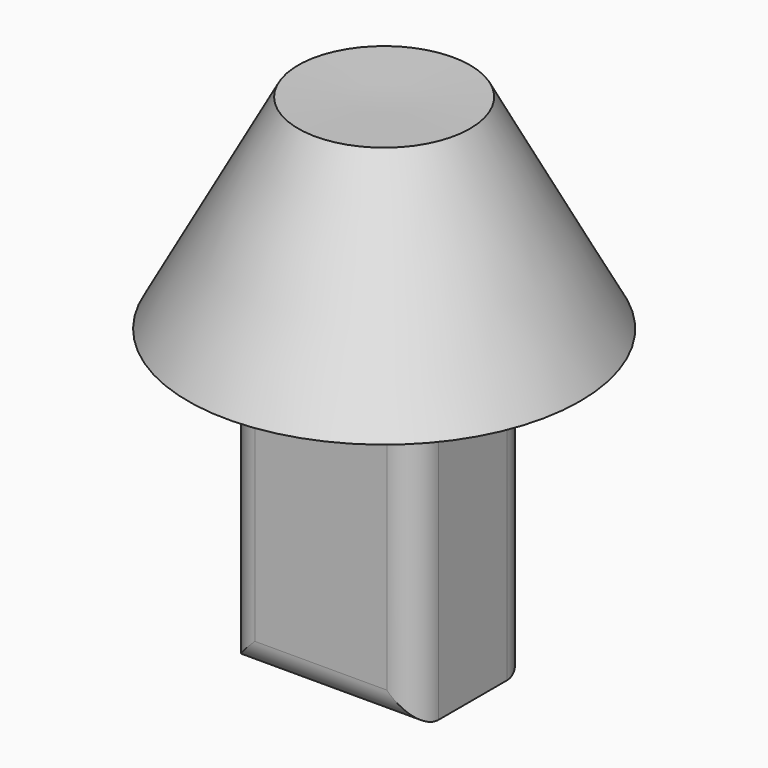
from build123d import *

# Parameters (mm, degrees)
F2_W         = 33.0171785317
F2_H         = 49.6530286036
F3_DEPTH     = 12.5
F4_R         = 5
F5_R         = 5
F6_T1_DEPTH  = 57.1530286036
F6_T3_DEPTH  = 58.0171785317
F6_T5_DEPTH  = 15
F6_S9_W      = 5
F6_S9_H      = 5
F6_T10_DEPTH = 5
F6_S15_W     = 5
F6_S15_H     = 5
F6_T16_DEPTH = 5
F6_T20_ANGLE = 90
F6_T22_ANGLE = 90


# Not quite as in the source:
# - a fillet or chamfer that OpenCascade refuses, or shapes differently, is made with other operations: its cross-section is extruded or revolved along the edge and cut away or added


with BuildPart() as f1:
    # F0 (on Front) → F1 (revolve)
    with BuildSketch(Plane.XZ):
        Polygon((10.2449354299, 42.7789126646), (10.2449354299, 7.6398269811), (44.4469846271, 7.6398269811), (25.2376164656, 43.2474373302), align=None)
    revolve(axis=Axis((10.2449354299, 0, 25.2093698228), (0, 0, 1)))


with BuildPart() as f3:
    # F2 (on Front) → F3 (new body, symmetric)
    with BuildSketch(Plane.XZ):
        with Locations((9.1960497666, -19.5281591732)):
            Rectangle(F2_W, F2_H)
    extrude(amount=F3_DEPTH, both=True)

    # F4
    f4_edges = [f3.edges().sort_by_distance(p)[0] for p in [
        (9.19605, 12.5, 5.298355),
    ]]
    fillet(f4_edges, radius=F4_R)

    # F5
    f5_edges = [f3.edges().sort_by_distance(p)[0] for p in [
        (9.19605, -12.5, 5.298355),
        (-7.312539, -12.5, -19.528159),
        (9.19605, -12.5, -44.354673),
        (25.704639, -12.5, -19.528159),
    ]]
    fillet(f5_edges, radius=F5_R)

    # F6: fillet of radius 5 on 4 edges, made by hand

    # F6_s2 → F6_t1 (cut)
    with BuildSketch(Plane.XY.offset(-56.854673475)):
        with BuildLine():
            ThreePointArc((-7.3125394993, 7.5), (-5.8480734052, 11.0355339059), (-2.3125394993, 12.5))
            Line((-2.3125394993, 12.5), (-7.3125394993, 12.5))
            Line((-7.3125394993, 12.5), (-7.3125394993, 7.5))
        make_face()
        with BuildLine():
            ThreePointArc((25.7046390325, 7.5), (24.2401729384, 11.0355339059), (20.7046390325, 12.5))
            Line((20.7046390325, 12.5), (25.7046390325, 12.5))
            Line((25.7046390325, 12.5), (25.7046390325, 7.5))
        make_face()
    extrude(amount=F6_T1_DEPTH, mode=Mode.SUBTRACT)

    # F6_s4 → F6_t3 (cut)
    with BuildSketch(Plane.YZ.offset(-19.8125394993)):
        with BuildLine():
            ThreePointArc((7.5, -44.354673475), (11.0355339059, -42.890207381), (12.5, -39.354673475))
            Line((12.5, -39.354673475), (12.5, -44.354673475))
            Line((12.5, -44.354673475), (7.5, -44.354673475))
        make_face()
    extrude(amount=F6_T3_DEPTH, mode=Mode.SUBTRACT)

    # F6_s6 → F6_t5 (cut)
    with BuildSketch(Plane.XZ.offset(-7.5)):
        with BuildLine():
            ThreePointArc((20.7046390325, 5.2983551286), (24.2401729384, 3.8338890345), (25.7046390325, 0.2983551286))
            Line((25.7046390325, 0.2983551286), (25.7046390325, 5.2983551286))
            Line((25.7046390325, 5.2983551286), (20.7046390325, 5.2983551286))
        make_face()
        with BuildLine():
            ThreePointArc((-2.3125394993, 5.2983551286), (-5.8480734052, 3.8338890345), (-7.3125394993, 0.2983551286))
            Line((-7.3125394993, 0.2983551286), (-7.3125394993, 5.2983551286))
            Line((-7.3125394993, 5.2983551286), (-2.3125394993, 5.2983551286))
        make_face()
    extrude(amount=F6_T5_DEPTH, mode=Mode.SUBTRACT)


with BuildPart() as f6_tool8:
    # F6_s9 → F6_t10 (new body)
    with BuildSketch(Plane.XY.offset(0.2983551286)):
        with Locations((23.2046390325, -10)):
            Rectangle(F6_S9_W, F6_S9_H)
    extrude(amount=F6_T10_DEPTH)

    # F6_s11 → F6_t12 (revolve, cut)
    with BuildSketch(Plane(origin=(20.7046390325, -7.5, 0.2983551286), x_dir=(-0.7071067812, 0.7071067812, 0), z_dir=(0.7071067812, 0.7071067812, 0))):
        with BuildLine():
            ThreePointArc((0, -5), (5, 0), (0, 5))
            Line((0, 5), (0, -5))
        make_face()
    revolve(axis=Axis((20.7046390325, -7.5, 0.2983551286), (0, 0, 1)), mode=Mode.SUBTRACT)


with BuildPart() as f3_1:
    add(f3.part)

    # F6_t7: cut F6_tool8
    add(f6_tool8.part, mode=Mode.SUBTRACT)


with BuildPart() as f6_tool14:
    # F6_s15 → F6_t16 (new body)
    with BuildSketch(Plane.XY.offset(0.2983551286)):
        with Locations((-4.8125394993, -10)):
            Rectangle(F6_S15_W, F6_S15_H)
    extrude(amount=F6_T16_DEPTH)

    # F6_s17 → F6_t18 (revolve, cut)
    with BuildSketch(Plane(origin=(-2.3125394993, -7.5, 0.2983551286), x_dir=(0.7071067812, 0.7071067812, 0), z_dir=(0.7071067812, -0.7071067812, 0))):
        with BuildLine():
            ThreePointArc((0, -5), (5, 0), (0, 5))
            Line((0, 5), (0, -5))
        make_face()
    revolve(axis=Axis((-2.3125394993, -7.5, 0.2983551286), (0, 0, 1)), mode=Mode.SUBTRACT)


with BuildPart() as f3_2:
    add(f3_1.part)

    # F6_t13: cut F6_tool14
    add(f6_tool14.part, mode=Mode.SUBTRACT)

    # F6_s19 → F6_t20 (revolve, cut)
    with BuildSketch(Plane.XZ.offset(-7.5)):
        with BuildLine():
            ThreePointArc((20.7046390325, 5.2983551286), (24.2401729384, 3.8338890345), (25.7046390325, 0.2983551286))
            Line((25.7046390325, 0.2983551286), (25.7046390325, 5.2983551286))
            Line((25.7046390325, 5.2983551286), (20.7046390325, 5.2983551286))
        make_face()
    revolve(axis=Axis((25.7046390325, 7.5, 0.2983551286), (-1, 0, 0)), revolution_arc=F6_T20_ANGLE, mode=Mode.SUBTRACT)

    # F6_s21 → F6_t22 (revolve, cut)
    with BuildSketch(Plane.XZ.offset(-7.5)):
        with BuildLine():
            ThreePointArc((-7.3125394993, 0.2983551286), (-5.8480734052, 3.8338890345), (-2.3125394993, 5.2983551286))
            Line((-2.3125394993, 5.2983551286), (-7.3125394993, 5.2983551286))
            Line((-7.3125394993, 5.2983551286), (-7.3125394993, 0.2983551286))
        make_face()
    revolve(axis=Axis((-7.3125394993, 7.5, 0.2983551286), (-1, 0, 0)), revolution_arc=F6_T22_ANGLE, mode=Mode.SUBTRACT)


solid = Compound([f1.part, f3_2.part])
